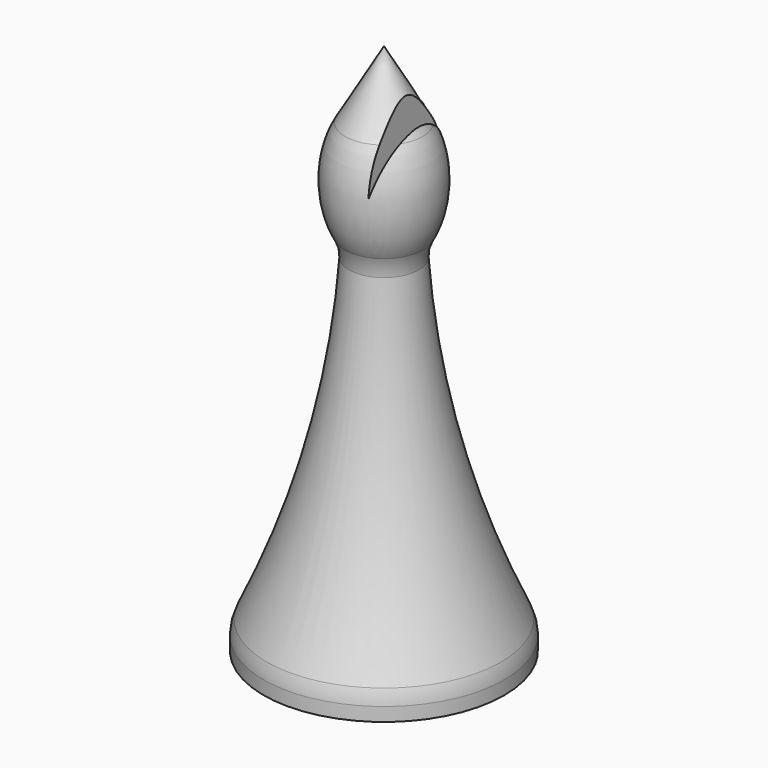
from build123d import *

# Parameters (mm, degrees)
F3_DEPTH = 12.7
F4_R     = 5.08


with BuildPart() as f1:
    # F0 (on Front) → F1 (revolve)
    with BuildSketch(Plane.XZ):
        with BuildLine():
            Line((-17.907, 3.175), (-17.907, 0))
            Line((-17.907, 0), (-8.636, 0))
            Line((-8.636, 0), (-8.636, 6.604))
            Line((-8.636, 6.604), (-5.1435, 10.0965))
            Line((-5.1435, 10.0965), (-5.1435, 31.75))
            Line((-5.1435, 31.75), (0, 36.8935))
            Line((0, 36.8935), (0, 79.248))
            Line((0, 79.248), (-5.7601785687, 69.2710780584))
            add(Edge.make_bspline(
                [(-5.7601785687, 69.2710780584), (-10.6664197671, 60.7732190285), (-5.0834936393, 53.2736577196)],
                knots=[0.8570719479, 0.8570719479, 0.8570719479, 2.4112497087, 2.4112497087, 2.4112497087], degree=2, weights=[1, 0.7129578532, 1]))
            ThreePointArc((-5.0834936393, 53.2736577196), (-9.0107667422, 27.5883887463), (-17.907, 3.175))
        make_face()
    revolve(axis=Axis((0, 0, 18.44675), (0, 0, -1)))

    # F2 (on Front) → F3 (cut, symmetric)
    with BuildSketch(Plane.XZ):
        Polygon((7.2810413163, 78.2450328688), (3.175, 79.0126742409), (3.175, 62.9210780584), align=None)
    extrude(amount=F3_DEPTH, both=True, mode=Mode.SUBTRACT)

    # F4
    f4_edges = [f1.edges().sort_by_distance(p)[0] for p in [
        (5.083494, 0, 53.273658),
        (17.907, 0, 3.175),
    ]]
    fillet(f4_edges, radius=F4_R)


solid = f1.part
